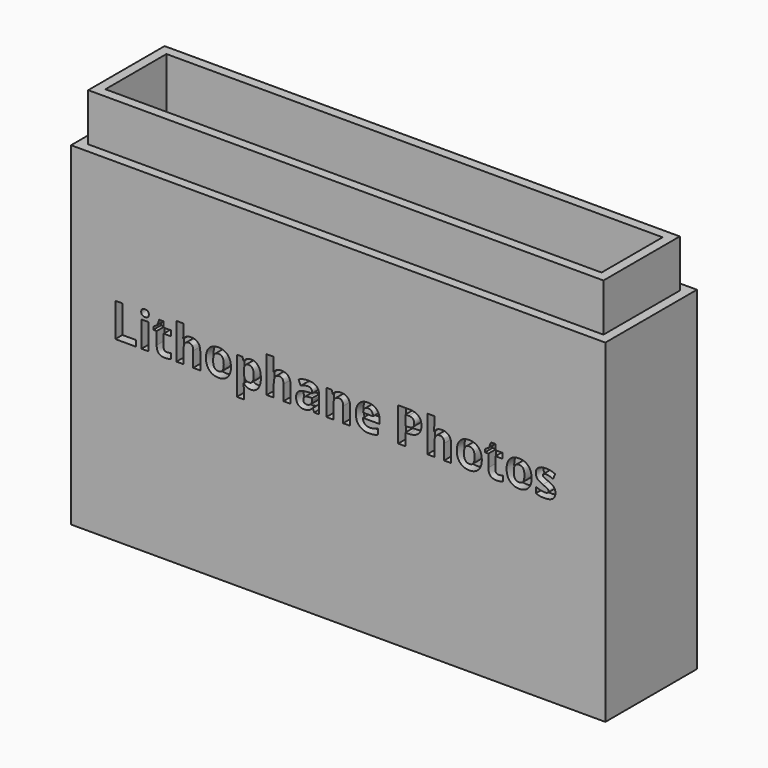
from build123d import *

# Parameters (mm, degrees)
F0_W         = 112
F0_H         = 24
F1_DEPTH     = 80
F2_W         = 104
F2_H         = 16
F3_DEPTH     = 78
F4_W         = 112
F4_H         = 24
F4_W_2       = 108
F4_H_2       = 20
F5_DEPTH     = 10
F6_TEXT_SIZE = 9.9097792473
F7_DEPTH     = 2


# Not quite as in the source:
# - Text() gives the source's letters only with a copy of the font that has no kerning and outlines rounded to 1/6400 em; it was checked with that copy


with BuildPart() as f1:
    # F0 (on Top) → F1 (new body)
    with BuildSketch(Plane.XY):
        with Locations((51.61290384, 7.9879021719)):
            Rectangle(F0_W, F0_H)
    extrude(amount=F1_DEPTH)

    # F2 (on face) → F3 (cut)
    with BuildSketch(Plane.XY.offset(80)):
        with Locations((51.61290384, 7.9879021719)):
            Rectangle(F2_W, F2_H)
    extrude(amount=-F3_DEPTH, mode=Mode.SUBTRACT)

    # F4 (on face) → F5 (cut)
    with BuildSketch(Plane.XY.offset(80)):
        with Locations((51.61290384, 7.9879021719)):
            Rectangle(F4_W, F4_H)
        with Locations((51.61290384, 7.9879021719)):
            Rectangle(F4_W_2, F4_H_2, mode=Mode.SUBTRACT)
    extrude(amount=-F5_DEPTH, mode=Mode.SUBTRACT)

    # F6 (on face) → F7 (cut)
    with BuildSketch(Plane.XZ.offset(4.0120978281)):
        with Locations((4.00519697, 37.2435413301)):
            Text('Lithophane Photos', F6_TEXT_SIZE, font='Open Sans', font_style=FontStyle.BOLD, text_align=(TextAlign.LEFT, TextAlign.BOTTOM))
    extrude(amount=-F7_DEPTH, mode=Mode.SUBTRACT)


solid = f1.part
